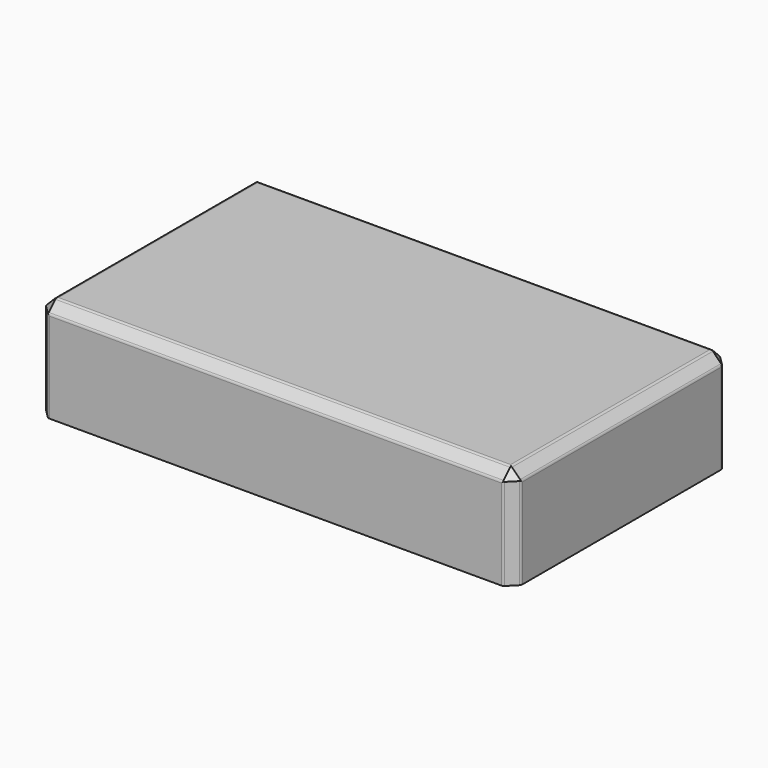
from build123d import *

# Parameters (mm, degrees)
F0_W        = 140
F0_H        = 80
F1_DEPTH    = 30
F2_SIZE     = 3
F3_T1_DEPTH = 29.0710678119
F3_T3_DEPTH = 136.0710678119
F3_T5_DEPTH = 76.0710678119


# Not quite as in the source:
# - a fillet or chamfer that OpenCascade refuses, or shapes differently, is made with other operations: its cross-section is extruded or revolved along the edge and cut away or added


with BuildPart() as f1:
    # F0 (on Top) → F1 (new body)
    with BuildSketch(Plane.XY):
        Rectangle(F0_W, F0_H)
    extrude(amount=F1_DEPTH)

    # F2
    f2_edges = [f1.edges().sort_by_distance(p)[0] for p in [
        (0, -40, 30),
        (-70, 0, 30),
        (0, 40, 30),
        (70, 0, 30),
        (70, -40, 15),
        (-70, -40, 15),
        (-70, 40, 15),
        (70, 40, 15),
    ]]
    chamfer(f2_edges, length=F2_SIZE)

    # F3: fillet of radius 1 on 16 edges, made by hand

    # F3_s2 → F3_t1 (cut)
    with BuildSketch(Plane.XY.offset(-1.0355339059)):
        with BuildLine():
            ThreePointArc((70, 36.5857864376), (69.9238795325, 36.96846987), (69.7071067812, 37.2928932188))
            Line((69.7071067812, 37.2928932188), (70, 37))
            Line((70, 37), (70, 36.5857864376))
        make_face()
        with BuildLine():
            ThreePointArc((67.2928932188, 39.7071067812), (66.96846987, 39.9238795325), (66.5857864376, 40))
            Line((66.5857864376, 40), (67, 40))
            Line((67, 40), (67.2928932188, 39.7071067812))
        make_face()
        with BuildLine():
            ThreePointArc((-67.2928932188, 39.7071067812), (-66.96846987, 39.9238795325), (-66.5857864376, 40))
            Line((-66.5857864376, 40), (-67, 40))
            Line((-67, 40), (-67.2928932188, 39.7071067812))
        make_face()
        with BuildLine():
            ThreePointArc((-70, 36.5857864376), (-69.9238795325, 36.96846987), (-69.7071067812, 37.2928932188))
            Line((-69.7071067812, 37.2928932188), (-70, 37))
            Line((-70, 37), (-70, 36.5857864376))
        make_face()
        with BuildLine():
            ThreePointArc((69.7071067812, -37.2928932188), (69.9238795325, -36.96846987), (70, -36.5857864376))
            Line((70, -36.5857864376), (70, -37))
            Line((70, -37), (69.7071067812, -37.2928932188))
        make_face()
        with BuildLine():
            ThreePointArc((66.5857864376, -40), (66.96846987, -39.9238795325), (67.2928932188, -39.7071067812))
            Line((67.2928932188, -39.7071067812), (67, -40))
            Line((67, -40), (66.5857864376, -40))
        make_face()
        with BuildLine():
            ThreePointArc((-69.7071067812, -37.2928932188), (-69.9238795325, -36.96846987), (-70, -36.5857864376))
            Line((-70, -36.5857864376), (-70, -37))
            Line((-70, -37), (-69.7071067812, -37.2928932188))
        make_face()
        with BuildLine():
            ThreePointArc((-66.5857864376, -40), (-66.96846987, -39.9238795325), (-67.2928932188, -39.7071067812))
            Line((-67.2928932188, -39.7071067812), (-67, -40))
            Line((-67, -40), (-66.5857864376, -40))
        make_face()
    extrude(amount=F3_T1_DEPTH, mode=Mode.SUBTRACT)

    # F3_s4 → F3_t3 (cut)
    with BuildSketch(Plane.YZ.offset(-68.0355339059)):
        with BuildLine():
            ThreePointArc((40, 26.5857864376), (39.9238795325, 26.96846987), (39.7071067812, 27.2928932188))
            Line((39.7071067812, 27.2928932188), (40, 27))
            Line((40, 27), (40, 26.5857864376))
        make_face()
        with BuildLine():
            ThreePointArc((36.5857864376, 30), (36.96846987, 29.9238795325), (37.2928932188, 29.7071067812))
            Line((37.2928932188, 29.7071067812), (37, 30))
            Line((37, 30), (36.5857864376, 30))
        make_face()
        with BuildLine():
            ThreePointArc((-37.2928932188, 29.7071067812), (-36.96846987, 29.9238795325), (-36.5857864376, 30))
            Line((-36.5857864376, 30), (-37, 30))
            Line((-37, 30), (-37.2928932188, 29.7071067812))
        make_face()
        with BuildLine():
            ThreePointArc((-40, 26.5857864376), (-39.9238795325, 26.96846987), (-39.7071067812, 27.2928932188))
            Line((-39.7071067812, 27.2928932188), (-40, 27))
            Line((-40, 27), (-40, 26.5857864376))
        make_face()
    extrude(amount=F3_T3_DEPTH, mode=Mode.SUBTRACT)

    # F3_s6 → F3_t5 (cut)
    with BuildSketch(Plane.XZ.offset(-38.0355339059)):
        with BuildLine():
            ThreePointArc((66.5857864376, 30), (66.96846987, 29.9238795325), (67.2928932188, 29.7071067812))
            Line((67.2928932188, 29.7071067812), (67, 30))
            Line((67, 30), (66.5857864376, 30))
        make_face()
        with BuildLine():
            ThreePointArc((70, 26.5857864376), (69.9238795325, 26.96846987), (69.7071067812, 27.2928932188))
            Line((69.7071067812, 27.2928932188), (70, 27))
            Line((70, 27), (70, 26.5857864376))
        make_face()
        with BuildLine():
            ThreePointArc((-66.5857864376, 30), (-66.96846987, 29.9238795325), (-67.2928932188, 29.7071067812))
            Line((-67.2928932188, 29.7071067812), (-67, 30))
            Line((-67, 30), (-66.5857864376, 30))
        make_face()
        with BuildLine():
            ThreePointArc((-70, 26.5857864376), (-69.9238795325, 26.96846987), (-69.7071067812, 27.2928932188))
            Line((-69.7071067812, 27.2928932188), (-70, 27))
            Line((-70, 27), (-70, 26.5857864376))
        make_face()
    extrude(amount=F3_T5_DEPTH, mode=Mode.SUBTRACT)


solid = f1.part
